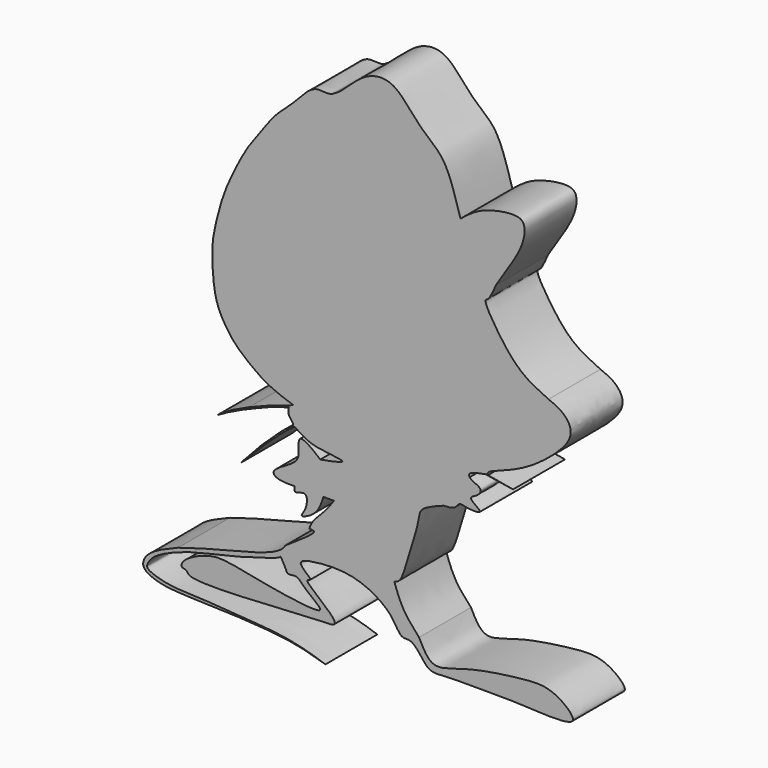
from build123d import *

# Parameters (mm, degrees)
F1_DEPTH = 3
F2_DEPTH = 3
F3_DEPTH = 3


with BuildPart() as f1:
    # F0 (on Front) → F1 (new body)
    with BuildSketch(Plane.XZ):
        with BuildLine():
            add(Edge.make_bspline(
                [(3.4387107007, -3.7845890038), (3.6329386245, -3.7760784632), (3.9740611591, -3.7611313994), (4.1446707489, -3.43705762), (4.3718387119, -3.4856108812), (4.6012481057, -3.5448908247), (5.443142395, -3.5558585306), (4.4833661791, -3.0685286694), (4.9663246867, -2.921390953), (5.3367543683, -2.4983211696), (4.7792190937, -2.3785138693), (4.6374006197, -2.2387674544)],
                knots=[0, 0, 0, 0, 0.0544068628, 0.0955547821, 0.1272545557, 0.1690446021, 0.2205523866, 0.2769745476, 0.3185512029, 0.365204984, 0.4237224473, 0.4237224473, 0.4237224473, 0.4237224473], degree=3))
            add(Edge.make_bspline(
                [(4.6374006197, -2.2387674544), (4.5010791837, -2.1044377623), (4.5420444151, -1.675366264), (4.9437050845, -1.0420811512), (4.794231832, -0.8718639546), (3.6699129493, -1.1863080631), (3.6239571551, -1.725744032), (3.262399267, -1.5549323864), (3.0435898188, -1.9790971235), (1.6708210432, -2.3726101816), (1.9018707979, -3.0488359763), (1.2028652444, -3.442513783), (0.77228999, -3.6850124598)],
                knots=[0.4237224473, 0.4237224473, 0.4237224473, 0.4237224473, 0.4799717102, 0.5432857754, 0.5692996053, 0.6471112563, 0.6950420399, 0.7316574761, 0.7805713207, 0.8651463027, 0.9169324696, 1, 1, 1, 1], degree=3))
            add(Edge.make_bspline(
                [(0.77228999, -3.6850124598), (0.6268164852, -3.7706924059), (0.3253982077, -3.9482195909), (0.1833538063, -3.2408059574), (-0.1852659269, -3.582603144), (-0.827380499, -3.5323231042), (-1.2483170722, -3.4993621521)],
                knots=[0, 0, 0, 0, 0.2177106419, 0.4510922232, 0.6401649042, 1, 1, 1, 1], degree=3))
            add(Edge.make_bspline(
                [(-1.2483170722, -3.4993621521), (-1.2021052852, -3.5685746762), (-1.7337150506, -3.665539381), (-2.2653248161, -3.7625040859)],
                knots=[0.7185690783, 0.7185690783, 0.7185690783, 0.7185690783, 1, 1, 1, 1], degree=3))
            add(Edge.make_bspline(
                [(-2.2653248161, -3.7625040859), (-2.364691852, -3.67330553), (-2.5780364083, -3.4817930614), (-3.3739941303, -2.9603068835), (-3.1790482255, -3.9862522573), (-3.5360105307, -4.3778604471), (-4.5657746047, -4.8788945221), (-4.2821051876, -5.2392585433), (-3.7844307871, -5.236484235), (-3.4601313528, -5.2346764132)],
                knots=[0, 0, 0, 0, 0.1256561107, 0.2697881339, 0.4200930903, 0.5605554978, 0.7427142556, 0.8323449603, 1, 1, 1, 1], degree=3))
            add(Edge.make_bspline(
                [(-3.4601313528, -5.2346764132), (-3.4670770018, -5.3360046299), (-3.4836193946, -5.5773371758), (-2.8418900026, -5.1890090468), (-2.8657727929, -5.986474129), (-3.3026190577, -6.4592858538), (-2.5410436163, -6.1420571651), (-2.2365569591, -5.6325547263), (-2.1577624363, -5.3562669771), (-2.1230860148, -5.2346764132)],
                knots=[0, 0, 0, 0, 0.101598322, 0.2419758536, 0.4043293397, 0.5396333121, 0.6936217106, 0.8651669897, 1, 1, 1, 1], degree=3))
            add(Edge.make_bspline(
                [(-2.1230860148, -5.2346764132), (-1.9602796528, -5.2346764132), (-1.7974732909, -5.2346764132), (-1.634666929, -5.2346764132)],
                knots=[0, 0, 0, 0, 0.4884190857, 0.4884190857, 0.4884190857, 0.4884190857], degree=3))
            add(Edge.make_bspline(
                [(-1.634666929, -5.2346764132), (-1.7588757926, -5.4176151051), (-2.0173616645, -5.7983211666), (-2.632941209, -6.3525404519), (-2.731008143, -6.627434248), (-2.7711989824, -6.7400941625)],
                knots=[0, 0, 0, 0, 0.3531352326, 0.7348949652, 1, 1, 1, 1], degree=3))
            add(Edge.make_bspline(
                [(-2.7711989824, -6.7400941625), (-2.6686582403, -6.7431192559), (-2.5661174981, -6.7461443493), (-2.5599850342, -6.7903832532)],
                knots=[0, 0, 0, 0, 0.2047211831, 0.2047211831, 0.2047211831, 0.2047211831], degree=3))
            add(Edge.make_bspline(
                [(1.1555887759, -7.6065552421), (0.8608182174, -7.6838857733), (0.2812095174, -7.8359411514), (-0.5809110342, -7.8263457193), (-1.6414123271, -7.2404493989), (-2.2608775483, -6.9369346936), (-2.5599850342, -6.7903832532)],
                knots=[0, 0, 0, 0, 0.2385009214, 0.4689654549, 0.7435910811, 1, 1, 1, 1], degree=3))
            add(Edge.make_bspline(
                [(1.1555887759, -7.6065552421), (1.2383360169, -7.5905019221), (1.4971560383, -7.5402897269), (1.8158186358, -6.2776181207), (2.1678735901, -5.2862975684), (2.3044200083, -4.6198026027), (2.3808646804, -4.1818000984), (3.0286826706, -3.9385506197), (3.4387107007, -3.7845890038)],
                knots=[0, 0, 0, 0, 0.1006764661, 0.3148997452, 0.5232921898, 0.6785016722, 0.7965117857, 1, 1, 1, 1], degree=3))
        make_face()
        with BuildLine():
            add(Edge.make_bspline(
                [(5.4890182801, -1.8760111416), (5.4763511637, -1.8431545871), (5.4196371221, -1.6960470732), (6.8179546909, -1.2881565459), (7.8569903576, -0.6238466356), (8.4862095822, -0.0866460392), (8.5815473163, 0)],
                knots=[0, 0, 0, 0, 0.0541533604, 0.2424589657, 0.4808610331, 0.5253393727, 0.5253393727, 0.5253393727, 0.5253393727], degree=3))
            Line((8.5815473163, 0), (-6.4611709528, 0))
            add(Edge.make_bspline(
                [(-6.4611709528, 0), (-6.4216262025, -0.0558948523), (-6.3816453943, -0.1116198328), (-6.3416645862, -0.1673448132)],
                knots=[0.9718688618, 0.9718688618, 0.9718688618, 0.9718688618, 1, 1, 1, 1], degree=3))
            add(Edge.make_bspline(
                [(-6.3416645862, -0.1673448132), (-6.2151357341, -0.3085234172), (-5.9412669679, -0.6141012317), (-5.2859553373, -1.1068613012), (-4.8118201589, -1.4343205117), (-4.2246778477, -1.708310116), (-3.7580800733, -1.8677393367), (-3.5140283871, -1.9511280116)],
                knots=[0, 0, 0, 0, 0.1885814346, 0.4081801419, 0.5941253751, 0.7877092606, 1, 1, 1, 1], degree=3))
            add(Edge.make_bspline(
                [(-3.5140283871, -1.9511280116), (-3.6223852715, -1.9964466958), (-3.8468265168, -2.0903159685), (-4.2295321785, -2.1850227392), (-5.0008918764, -2.4724189651), (-5.3778256371, -2.6281814057), (-5.5522238836, -2.700248966)],
                knots=[0, 0, 0, 0, 0.2030129044, 0.4205036841, 0.7318808983, 1, 1, 1, 1], degree=3))
            add(Edge.make_bspline(
                [(-5.5522238836, -2.700248966), (-5.6810285383, -2.7604108896), (-5.9512230069, -2.8866129978), (-6.3174605139, -3.026516728), (-7.3719013529, -3.7175880069), (-6.2511121814, -3.0449710833), (-5.5217121999, -2.7801067023), (-4.6670381406, -2.376040331), (-4.0372573418, -2.2012844898), (-3.7152133882, -2.1119215526)],
                knots=[0, 0, 0, 0, 0.1073218681, 0.2251298695, 0.3693644548, 0.5127381771, 0.6741963054, 0.8333974137, 1, 1, 1, 1], degree=3))
            add(Edge.make_bspline(
                [(-3.7152133882, -2.1119215526), (-3.7392498379, -2.2120576332), (-3.7904079402, -2.4251827791), (-3.382741716, -2.7808957122), (-3.8281313937, -2.9532305527), (-4.4297151847, -3.5577305778), (-5.0385534929, -4.0940590889), (-5.4740909647, -4.596828966), (-6.2317515154, -5.3941615245), (-5.2563859558, -4.3849942527), (-4.6750627269, -3.8558362622), (-3.9524911135, -3.169717552), (-3.6111368003, -2.924911061), (-3.4601313528, -2.8166156262)],
                knots=[0, 0, 0, 0, 0.0621327088, 0.1322404726, 0.1956877793, 0.3014409733, 0.4024621197, 0.5019658908, 0.5883960501, 0.6924830371, 0.8036519499, 0.9131412024, 1, 1, 1, 1], degree=3))
            add(Edge.make_bspline(
                [(-3.4601313528, -2.8166156262), (-3.2969439654, -2.9171923914), (-2.9574505408, -3.1264312975), (-2.4796507396, -3.353661953), (-1.2964318583, -3.4272994596), (-1.2483170722, -3.4993621521)],
                knots=[0, 0, 0, 0, 0.2045524277, 0.4255488447, 0.7185690783, 0.7185690783, 0.7185690783, 0.7185690783], degree=3))
            add(Edge.make_bspline(
                [(0.77228999, -3.6850124598), (0.6268164852, -3.7706924059), (0.3253982077, -3.9482195909), (0.1833538063, -3.2408059574), (-0.1852659269, -3.582603144), (-0.827380499, -3.5323231042), (-1.2483170722, -3.4993621521)],
                knots=[0, 0, 0, 0, 0.2177106419, 0.4510922232, 0.6401649042, 1, 1, 1, 1], degree=3))
            add(Edge.make_bspline(
                [(4.6374006197, -2.2387674544), (4.5010791837, -2.1044377623), (4.5420444151, -1.675366264), (4.9437050845, -1.0420811512), (4.794231832, -0.8718639546), (3.6699129493, -1.1863080631), (3.6239571551, -1.725744032), (3.262399267, -1.5549323864), (3.0435898188, -1.9790971235), (1.6708210432, -2.3726101816), (1.9018707979, -3.0488359763), (1.2028652444, -3.442513783), (0.77228999, -3.6850124598)],
                knots=[0.4237224473, 0.4237224473, 0.4237224473, 0.4237224473, 0.4799717102, 0.5432857754, 0.5692996053, 0.6471112563, 0.6950420399, 0.7316574761, 0.7805713207, 0.8651463027, 0.9169324696, 1, 1, 1, 1], degree=3))
            add(Edge.make_bspline(
                [(4.6374006197, -2.2387674544), (4.6214342628, -2.1887250094), (4.5683139999, -2.022233188), (5.0453890142, -1.9361913708), (5.3790695965, -1.8760111416)],
                knots=[0, 0, 0, 0, 0.3005699893, 1, 1, 1, 1], degree=3))
            add(Edge.make_bspline(
                [(5.3790695965, -1.8760111416), (6.0131320281, -1.979027022), (7.2539084801, -2.1806154969), (6.0686064538, -1.9760429067), (5.4890182801, -1.8760111416)],
                knots=[0, 0, 0, 0, 0.5110206843, 1, 1, 1, 1], degree=3))
        make_face()
        with BuildLine():
            Line((-6.4611709528, 0), (8.5815473163, 0))
            add(Edge.make_bspline(
                [(8.5815473163, 0), (8.9542029485, 0.338681581), (9.5513763508, 1.0378960315), (8.993312318, 1.8440750015), (8.5207671535, 2.0320276216), (8.2884747535, 2.1244208328)],
                knots=[0.5253393727, 0.5253393727, 0.5253393727, 0.5253393727, 0.6991960717, 0.8521316655, 1, 1, 1, 1], degree=3))
            add(Edge.make_bspline(
                [(8.2884747535, 2.1244208328), (7.9048585922, 2.3025485753), (7.0975296441, 2.6774224659), (6.1840751164, 3.6842317456), (5.2260969843, 5.2162763203), (5.5500812962, 5.2658802737), (5.7315738672, 5.6877215628), (5.8569866233, 5.9792171232)],
                knots=[0, 0, 0, 0, 0.2297754545, 0.483567677, 0.738307483, 0.8191684672, 1, 1, 1, 1], degree=3))
            add(Edge.make_bspline(
                [(5.8569866233, 5.9792171232), (6.0931747194, 6.3363678983), (6.5640208915, 7.048355835), (7.1885956872, 8.1339473276), (7.2214251672, 9.0459287336), (6.5098494676, 9.1628966401), (5.1058403554, 8.8710770917), (4.5053916385, 8.382268127), (4.2215422727, 8.1511940807)],
                knots=[0, 0, 0, 0, 0.1857054916, 0.3702079879, 0.50903551, 0.6312788248, 0.8256949032, 1, 1, 1, 1], degree=3))
            add(Edge.make_bspline(
                [(-1.6546921106, 11.3283833048), (-1.1760800507, 11.5773979686), (-0.4252394327, 12.5762978868), (1.157598532, 12.9050172504), (2.2805095167, 11.1922888241), (3.6119445205, 10.4309384936), (3.9828484215, 8.8832528519), (4.2215422727, 8.1511940807)],
                knots=[0, 0, 0, 0, 0.2012932908, 0.3764910203, 0.5829871374, 0.7703648661, 1, 1, 1, 1], degree=3))
            add(Edge.make_bspline(
                [(-1.6546921106, 11.3283833048), (-1.8988738366, 11.1776419827), (-2.5515191275, 11.4916285169), (-3.4537264232, 10.3323889139), (-4.4027012496, 9.5936121152), (-4.9487060772, 8.7436287047), (-5.6124526702, 7.9219520547), (-5.9527370044, 7.2653172924), (-6.1304159462, 6.9233463146)],
                knots=[0, 0, 0, 0, 0.144083091, 0.3277219301, 0.5070094801, 0.6659250705, 0.8296518383, 1, 1, 1, 1], degree=3))
            add(Edge.make_bspline(
                [(-6.1304159462, 6.9233463146), (-6.313250136, 6.5550671305), (-6.6783986445, 5.8195559278), (-7.0165330163, 4.6371550678), (-7.3121064813, 3.3804811956), (-7.2315220891, 1.978761829), (-7.0405351136, 0.857721861), (-6.6473129371, 0.263103917), (-6.4611709528, 0)],
                knots=[0, 0, 0, 0, 0.1655302972, 0.3305899255, 0.5002121636, 0.6768262828, 0.839452148, 0.9718688618, 0.9718688618, 0.9718688618, 0.9718688618], degree=3))
        make_face()
    extrude(amount=F1_DEPTH)

    # F0 (on Front) → F2 (join)
    with BuildSketch(Plane.XZ):
        with BuildLine():
            Line((-6.4611709528, 0), (8.5815473163, 0))
            add(Edge.make_bspline(
                [(8.5815473163, 0), (8.9542029485, 0.338681581), (9.5513763508, 1.0378960315), (8.993312318, 1.8440750015), (8.5207671535, 2.0320276216), (8.2884747535, 2.1244208328)],
                knots=[0.5253393727, 0.5253393727, 0.5253393727, 0.5253393727, 0.6991960717, 0.8521316655, 1, 1, 1, 1], degree=3))
            add(Edge.make_bspline(
                [(8.2884747535, 2.1244208328), (7.9048585922, 2.3025485753), (7.0975296441, 2.6774224659), (6.1840751164, 3.6842317456), (5.2260969843, 5.2162763203), (5.5500812962, 5.2658802737), (5.7315738672, 5.6877215628), (5.8569866233, 5.9792171232)],
                knots=[0, 0, 0, 0, 0.2297754545, 0.483567677, 0.738307483, 0.8191684672, 1, 1, 1, 1], degree=3))
            add(Edge.make_bspline(
                [(5.8569866233, 5.9792171232), (6.0931747194, 6.3363678983), (6.5640208915, 7.048355835), (7.1885956872, 8.1339473276), (7.2214251672, 9.0459287336), (6.5098494676, 9.1628966401), (5.1058403554, 8.8710770917), (4.5053916385, 8.382268127), (4.2215422727, 8.1511940807)],
                knots=[0, 0, 0, 0, 0.1857054916, 0.3702079879, 0.50903551, 0.6312788248, 0.8256949032, 1, 1, 1, 1], degree=3))
            add(Edge.make_bspline(
                [(-1.6546921106, 11.3283833048), (-1.1760800507, 11.5773979686), (-0.4252394327, 12.5762978868), (1.157598532, 12.9050172504), (2.2805095167, 11.1922888241), (3.6119445205, 10.4309384936), (3.9828484215, 8.8832528519), (4.2215422727, 8.1511940807)],
                knots=[0, 0, 0, 0, 0.2012932908, 0.3764910203, 0.5829871374, 0.7703648661, 1, 1, 1, 1], degree=3))
            add(Edge.make_bspline(
                [(-1.6546921106, 11.3283833048), (-1.8988738366, 11.1776419827), (-2.5515191275, 11.4916285169), (-3.4537264232, 10.3323889139), (-4.4027012496, 9.5936121152), (-4.9487060772, 8.7436287047), (-5.6124526702, 7.9219520547), (-5.9527370044, 7.2653172924), (-6.1304159462, 6.9233463146)],
                knots=[0, 0, 0, 0, 0.144083091, 0.3277219301, 0.5070094801, 0.6659250705, 0.8296518383, 1, 1, 1, 1], degree=3))
            add(Edge.make_bspline(
                [(-6.1304159462, 6.9233463146), (-6.313250136, 6.5550671305), (-6.6783986445, 5.8195559278), (-7.0165330163, 4.6371550678), (-7.3121064813, 3.3804811956), (-7.2315220891, 1.978761829), (-7.0405351136, 0.857721861), (-6.6473129371, 0.263103917), (-6.4611709528, 0)],
                knots=[0, 0, 0, 0, 0.1655302972, 0.3305899255, 0.5002121636, 0.6768262828, 0.839452148, 0.9718688618, 0.9718688618, 0.9718688618, 0.9718688618], degree=3))
        make_face()
        with BuildLine():
            add(Edge.make_bspline(
                [(2.3041076493, -9.5131369308), (2.0514618179, -9.2403588727), (1.5424326004, -8.6907673729), (1.2851663778, -7.9697240428), (1.1555887759, -7.6065552421)],
                knots=[0, 0, 0, 0, 0.4963287425, 1, 1, 1, 1], degree=3))
            add(Edge.make_bspline(
                [(1.1555887759, -7.6065552421), (0.8608182174, -7.6838857733), (0.2812095174, -7.8359411514), (-0.5809110342, -7.8263457193), (-1.6414123271, -7.2404493989), (-2.2608775483, -6.9369346936), (-2.5599850342, -6.7903832532)],
                knots=[0, 0, 0, 0, 0.2385009214, 0.4689654549, 0.7435910811, 1, 1, 1, 1], degree=3))
            add(Edge.make_bspline(
                [(-2.5599850342, -6.7903832532), (-2.5484307184, -6.873734785), (-3.2302430975, -7.3472429984), (-3.650877926, -7.6302848911), (-3.8674997631, -7.7760480344)],
                knots=[0.2047211831, 0.2047211831, 0.2047211831, 0.2047211831, 0.5904410508, 1, 1, 1, 1], degree=3))
            add(Edge.make_bspline(
                [(-3.8674997631, -7.7760480344), (-3.935543247, -7.8686813126), (-4.0035867309, -7.9613145908), (-4.1303657927, -8.0514848232)],
                knots=[0, 0, 0, 0, 0.1389962306, 0.1389962306, 0.1389962306, 0.1389962306], degree=3))
            add(Edge.make_bspline(
                [(-4.1053644381, -8.2928538322), (-4.0797579824, -8.2292516999), (-4.1050618875, -8.1403682616), (-4.1303657927, -8.0514848232)],
                knots=[0.9782908538, 0.9782908538, 0.9782908538, 0.9782908538, 1, 1, 1, 1], degree=3))
            add(Edge.make_bspline(
                [(-4.1053644381, -8.2928538322), (-4.0121991092, -8.4459680031), (-3.8594946222, -8.6969328328), (-3.7972118085, -8.9647911391), (-3.3131993303, -8.7878058254), (-3.0278339598, -9.2712123634), (-1.7918240003, -10.0351272519), (-3.549130512, -9.8831287978), (-5.182653349, -9.5804334439), (-6.654756886, -9.2775714765), (-7.4503182721, -9.3001155088), (-8.5627180099, -9.7961106119), (-8.7587098254, -10.2627158238), (-8.3954867076, -10.2498938578), (-8.4377597155, -10.7088991667), (-3.7600231879, -10.3887000168), (-2.5870386307, -10.3413856981), (-2.1230860148, -10.3226713836)],
                knots=[0, 0, 0, 0, 0.0500289508, 0.0820009476, 0.1249942441, 0.1797069274, 0.2474822994, 0.3207800604, 0.42030599, 0.5055696472, 0.5702180366, 0.6481495807, 0.6883986985, 0.7221902945, 0.7543613408, 0.9028421152, 1, 1, 1, 1], degree=3))
            add(Edge.make_bspline(
                [(-2.1230860148, -10.3226713836), (-1.8827633925, -10.3225684282), (-1.3417234351, -10.3223366439), (-2.0829701904, -9.5752086919), (-3.0989228386, -8.8161085815), (-2.5146985704, -8.8392793874), (-3.5660825921, -8.1927039217), (-2.2794467499, -7.9583369212), (-0.9025250531, -7.9215810417), (0.3548944553, -8.4414337149), (1.1159392222, -9.0986403543), (1.4558189057, -9.8555150083), (1.9497945783, -9.6847880805), (2.2629358217, -10.0861290484), (2.4474950042, -10.3226713836)],
                knots=[0, 0, 0, 0, 0.0696731717, 0.1568556863, 0.2539453689, 0.2908896706, 0.3684929071, 0.4526158573, 0.5715836662, 0.6813296175, 0.7779349037, 0.8578641843, 0.9162279946, 1, 1, 1, 1], degree=3))
            add(Edge.make_bspline(
                [(2.4474950042, -10.3226713836), (2.5574797245, -10.4673813055), (2.8077851104, -10.7967149868), (3.7154247159, -10.6705198686), (5.4564420142, -10.7078453504), (6.2308374442, -10.7031758656), (6.5738102421, -10.7011077926)],
                knots=[0, 0, 0, 0, 0.1787569031, 0.4068184696, 0.7372852147, 1, 1, 1, 1], degree=3))
            add(Edge.make_bspline(
                [(6.5738102421, -10.7011077926), (6.5983592057, -10.6999095174), (6.7229803603, -10.6938265546), (8.5247623607, -10.8272247547), (9.8104090598, -10.6683481056), (8.4790495549, -9.5426361015), (7.02655786, -9.6320912916), (4.399119207, -10.0081704291), (2.8924314619, -10.692059578), (2.4921343398, -9.8899174027), (2.3041076493, -9.5131369308)],
                knots=[0, 0, 0, 0, 0.0382626797, 0.1942379073, 0.2993541961, 0.4197400182, 0.5610162044, 0.7479151117, 0.8815912364, 1, 1, 1, 1], degree=3))
        make_face()
        with BuildLine():
            add(Edge.make_bspline(
                [(-4.1053644381, -8.2928538322), (-4.0797579824, -8.2292516999), (-4.1050618875, -8.1403682616), (-4.1303657927, -8.0514848232)],
                knots=[0.9782908538, 0.9782908538, 0.9782908538, 0.9782908538, 1, 1, 1, 1], degree=3))
            add(Edge.make_bspline(
                [(-4.1303657927, -8.0514848232), (-4.3562997393, -8.2121778919), (-5.3138708238, -8.5670729246), (-7.3024006566, -9.0199543162), (-8.351909506, -9.3400364479), (-8.841233328, -9.4892717898)],
                knots=[0.1389962306, 0.1389962306, 0.1389962306, 0.1389962306, 0.3867024883, 0.7140556913, 1, 1, 1, 1], degree=3))
            add(Edge.make_bspline(
                [(-8.841233328, -9.4892717898), (-9.2639276161, -9.6607448655), (-9.980495633, -9.9514327817), (-10.4448007067, -10.4184151104), (-10.4846367101, -10.8606984456), (-9.97592031, -11.1275888624), (-9.1715740265, -11.324547648), (-7.0496669886, -11.3519296757), (-5.1949492319, -11.4449847902), (-3.309717029, -11.6006780821), (-1.4175658765, -12.2283513476), (-3.6337248131, -11.4600803581), (-5.861293017, -11.3699293825), (-7.8411314516, -11.1830320307), (-9.2224942874, -11.1982536769), (-10.1513521608, -10.8935085354), (-10.3227536831, -10.7074458705), (-10.1039404156, -10.3372573603), (-9.6381412708, -9.9713476857), (-8.2064842025, -9.4083258878), (-6.5100623214, -9.1034885621), (-4.5034716888, -8.5061421789), (-4.1368637217, -8.3710927584), (-4.1053644381, -8.2928538322)],
                knots=[0, 0, 0, 0, 0.0495126304, 0.0839357625, 0.1098908874, 0.1404518964, 0.1806734724, 0.2444014007, 0.3056344699, 0.3697236605, 0.4160706487, 0.4682131558, 0.5387516203, 0.6005568675, 0.6531447016, 0.6950490053, 0.7137982475, 0.7399365657, 0.7738005207, 0.8271211187, 0.8880892303, 0.9515857698, 0.9782908538, 0.9782908538, 0.9782908538, 0.9782908538], degree=3))
        make_face()
    extrude(amount=F2_DEPTH)

    # F0 (on Front) → F3 (join)
    with BuildSketch(Plane.XZ):
        with BuildLine():
            add(Edge.make_bspline(
                [(2.3041076493, -9.5131369308), (2.0514618179, -9.2403588727), (1.5424326004, -8.6907673729), (1.2851663778, -7.9697240428), (1.1555887759, -7.6065552421)],
                knots=[0, 0, 0, 0, 0.4963287425, 1, 1, 1, 1], degree=3))
            add(Edge.make_bspline(
                [(1.1555887759, -7.6065552421), (0.8608182174, -7.6838857733), (0.2812095174, -7.8359411514), (-0.5809110342, -7.8263457193), (-1.6414123271, -7.2404493989), (-2.2608775483, -6.9369346936), (-2.5599850342, -6.7903832532)],
                knots=[0, 0, 0, 0, 0.2385009214, 0.4689654549, 0.7435910811, 1, 1, 1, 1], degree=3))
            add(Edge.make_bspline(
                [(-2.5599850342, -6.7903832532), (-2.5484307184, -6.873734785), (-3.2302430975, -7.3472429984), (-3.650877926, -7.6302848911), (-3.8674997631, -7.7760480344)],
                knots=[0.2047211831, 0.2047211831, 0.2047211831, 0.2047211831, 0.5904410508, 1, 1, 1, 1], degree=3))
            add(Edge.make_bspline(
                [(-3.8674997631, -7.7760480344), (-3.935543247, -7.8686813126), (-4.0035867309, -7.9613145908), (-4.1303657927, -8.0514848232)],
                knots=[0, 0, 0, 0, 0.1389962306, 0.1389962306, 0.1389962306, 0.1389962306], degree=3))
            add(Edge.make_bspline(
                [(-4.1053644381, -8.2928538322), (-4.0797579824, -8.2292516999), (-4.1050618875, -8.1403682616), (-4.1303657927, -8.0514848232)],
                knots=[0.9782908538, 0.9782908538, 0.9782908538, 0.9782908538, 1, 1, 1, 1], degree=3))
            add(Edge.make_bspline(
                [(-4.1053644381, -8.2928538322), (-4.0121991092, -8.4459680031), (-3.8594946222, -8.6969328328), (-3.7972118085, -8.9647911391), (-3.3131993303, -8.7878058254), (-3.0278339598, -9.2712123634), (-1.7918240003, -10.0351272519), (-3.549130512, -9.8831287978), (-5.182653349, -9.5804334439), (-6.654756886, -9.2775714765), (-7.4503182721, -9.3001155088), (-8.5627180099, -9.7961106119), (-8.7587098254, -10.2627158238), (-8.3954867076, -10.2498938578), (-8.4377597155, -10.7088991667), (-3.7600231879, -10.3887000168), (-2.5870386307, -10.3413856981), (-2.1230860148, -10.3226713836)],
                knots=[0, 0, 0, 0, 0.0500289508, 0.0820009476, 0.1249942441, 0.1797069274, 0.2474822994, 0.3207800604, 0.42030599, 0.5055696472, 0.5702180366, 0.6481495807, 0.6883986985, 0.7221902945, 0.7543613408, 0.9028421152, 1, 1, 1, 1], degree=3))
            add(Edge.make_bspline(
                [(-2.1230860148, -10.3226713836), (-1.8827633925, -10.3225684282), (-1.3417234351, -10.3223366439), (-2.0829701904, -9.5752086919), (-3.0989228386, -8.8161085815), (-2.5146985704, -8.8392793874), (-3.5660825921, -8.1927039217), (-2.2794467499, -7.9583369212), (-0.9025250531, -7.9215810417), (0.3548944553, -8.4414337149), (1.1159392222, -9.0986403543), (1.4558189057, -9.8555150083), (1.9497945783, -9.6847880805), (2.2629358217, -10.0861290484), (2.4474950042, -10.3226713836)],
                knots=[0, 0, 0, 0, 0.0696731717, 0.1568556863, 0.2539453689, 0.2908896706, 0.3684929071, 0.4526158573, 0.5715836662, 0.6813296175, 0.7779349037, 0.8578641843, 0.9162279946, 1, 1, 1, 1], degree=3))
            add(Edge.make_bspline(
                [(2.4474950042, -10.3226713836), (2.5574797245, -10.4673813055), (2.8077851104, -10.7967149868), (3.7154247159, -10.6705198686), (5.4564420142, -10.7078453504), (6.2308374442, -10.7031758656), (6.5738102421, -10.7011077926)],
                knots=[0, 0, 0, 0, 0.1787569031, 0.4068184696, 0.7372852147, 1, 1, 1, 1], degree=3))
            add(Edge.make_bspline(
                [(6.5738102421, -10.7011077926), (6.5983592057, -10.6999095174), (6.7229803603, -10.6938265546), (8.5247623607, -10.8272247547), (9.8104090598, -10.6683481056), (8.4790495549, -9.5426361015), (7.02655786, -9.6320912916), (4.399119207, -10.0081704291), (2.8924314619, -10.692059578), (2.4921343398, -9.8899174027), (2.3041076493, -9.5131369308)],
                knots=[0, 0, 0, 0, 0.0382626797, 0.1942379073, 0.2993541961, 0.4197400182, 0.5610162044, 0.7479151117, 0.8815912364, 1, 1, 1, 1], degree=3))
        make_face()
    extrude(amount=F3_DEPTH)


solid = f1.part
